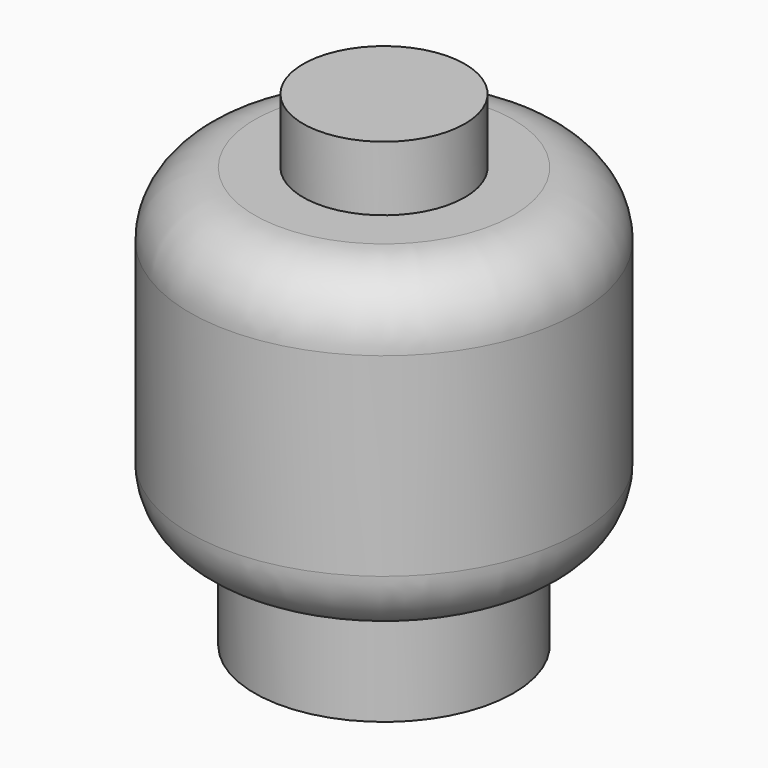
from build123d import *

# Parameters (mm, degrees)
F0_R     = 4
F1_DEPTH = 3
F2_R     = 6
F3_DEPTH = 10
F4_R     = 2.5
F5_DEPTH = 2
F6_R     = 2
F7_R     = 2.5
F8_DEPTH = 8


with BuildPart() as f1:
    # F0 (on Top) → F1 (new body)
    with BuildSketch(Plane.XY):
        Circle(F0_R)
    extrude(amount=F1_DEPTH)

    # F7 (on face) → F8 (cut)
    with BuildSketch(Plane(origin=(0, 0, 0), x_dir=(1, 0, 0), z_dir=(0, 0, -1))):
        Circle(F7_R)
    extrude(amount=-F8_DEPTH, mode=Mode.SUBTRACT)


with BuildPart() as f3:
    # F2 (on face) → F3 (new body)
    with BuildSketch(Plane.XY.offset(3)):
        Circle(F2_R)
    extrude(amount=F3_DEPTH)

    # F4 (on face) → F5 (join)
    with BuildSketch(Plane.XY.offset(13)):
        Circle(F4_R)
    extrude(amount=F5_DEPTH)

    # F6
    f6_edges = [f3.edges().sort_by_distance(p)[0] for p in [
        (-6, 0, 13),
        (-6, 0, 3),
    ]]
    fillet(f6_edges, radius=F6_R)


solid = Compound([f1.part, f3.part])
